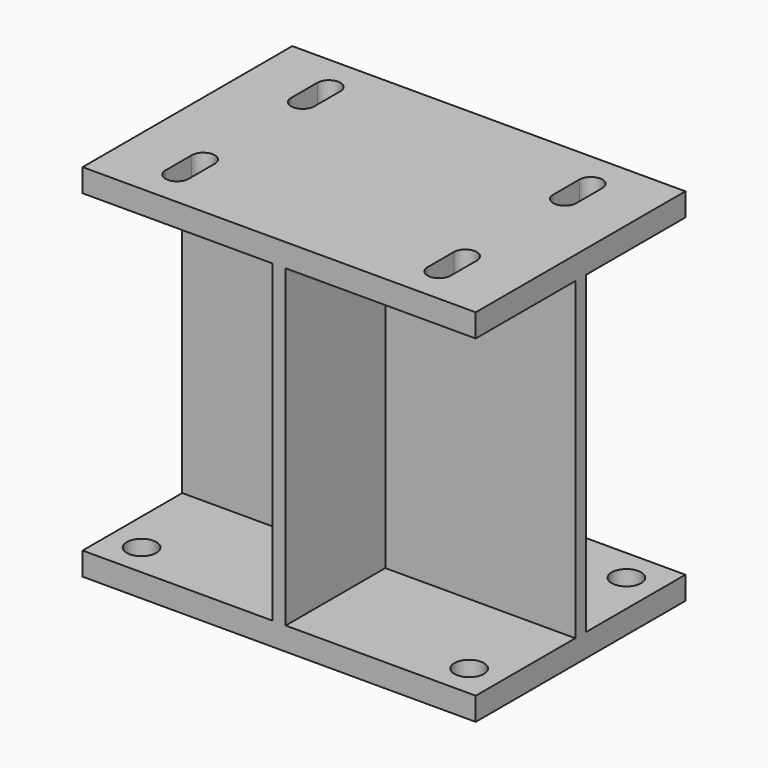
from build123d import *

# Parameters (mm, degrees)
F0_W     = 190.5
F0_H     = 127
F1_DEPTH = 11.176
F3_D     = 14.2875
F4_W     = 92.075
F4_H     = 6.35
F4_W_2   = 6.35
F4_H_2   = 60.325
F5_DEPTH = 152.4
F6_W     = 190.5
F6_H     = 127
F7_DEPTH = 11.176
F9_DEPTH = 25.4


# Not quite as in the source:
# - a length typed as a fraction of an inch, garbled in the dataset ("3 / 203.2 mm" for 3/8 in), is restored


with BuildPart() as f1:
    # F0 (on Top) → F1 (new body)
    with BuildSketch(Plane.XY):
        Rectangle(F0_W, F0_H)
    extrude(amount=F1_DEPTH)

    # F3 (through all)
    with Locations(Plane.XY.offset(11.176)):
        with Locations((-79.375, 47.625), (79.375, 47.625), (-79.375, -47.625), (79.375, -47.625)):
            Hole(F3_D / 2)

    # F4 (on face) → F5 (join)
    with BuildSketch(Plane.XY.offset(11.176)):
        with Locations((-49.2125, 0)):
            Rectangle(F4_W, F4_H)
        with Locations((0, 33.3375)):
            Rectangle(F4_W_2, F4_H_2)
        Rectangle(F4_W_2, F4_H)
        with Locations((49.2125, 0)):
            Rectangle(F4_W, F4_H)
        with Locations((0, -33.3375)):
            Rectangle(F4_W_2, F4_H_2)
    extrude(amount=F5_DEPTH)

    # F6 (on face) → F7 (join)
    with BuildSketch(Plane.XY.offset(163.576)):
        Rectangle(F6_W, F6_H)
    extrude(amount=F7_DEPTH)

    # F8 (on face) → F9 (cut)
    with BuildSketch(Plane.XY.offset(174.752)):
        with BuildLine():
            ThreePointArc((-69.088, -45.974), (-63.5, -51.562), (-57.912, -45.974))
            Line((-57.912, -45.974), (-57.912, -30.099))
            ThreePointArc((-57.912, -30.099), (-63.5, -24.511), (-69.088, -30.099))
            Line((-69.088, -30.099), (-69.088, -45.974))
        make_face()
        with BuildLine():
            Line((-57.912, 30.099), (-57.912, 45.974))
            ThreePointArc((-57.912, 45.974), (-63.5, 51.562), (-69.088, 45.974))
            Line((-69.088, 45.974), (-69.088, 30.099))
            ThreePointArc((-69.088, 30.099), (-63.5, 24.511), (-57.912, 30.099))
        make_face()
        with BuildLine():
            Line((69.088, 30.099), (69.088, 45.974))
            ThreePointArc((69.088, 45.974), (63.5, 51.562), (57.912, 45.974))
            Line((57.912, 45.974), (57.912, 30.099))
            ThreePointArc((57.912, 30.099), (63.5, 24.511), (69.088, 30.099))
        make_face()
        with BuildLine():
            Line((57.912, -30.099), (57.912, -45.974))
            ThreePointArc((57.912, -45.974), (63.5, -51.562), (69.088, -45.974))
            Line((69.088, -45.974), (69.088, -30.099))
            ThreePointArc((69.088, -30.099), (63.5, -24.511), (57.912, -30.099))
        make_face()
    extrude(amount=-F9_DEPTH, mode=Mode.SUBTRACT)


solid = f1.part
